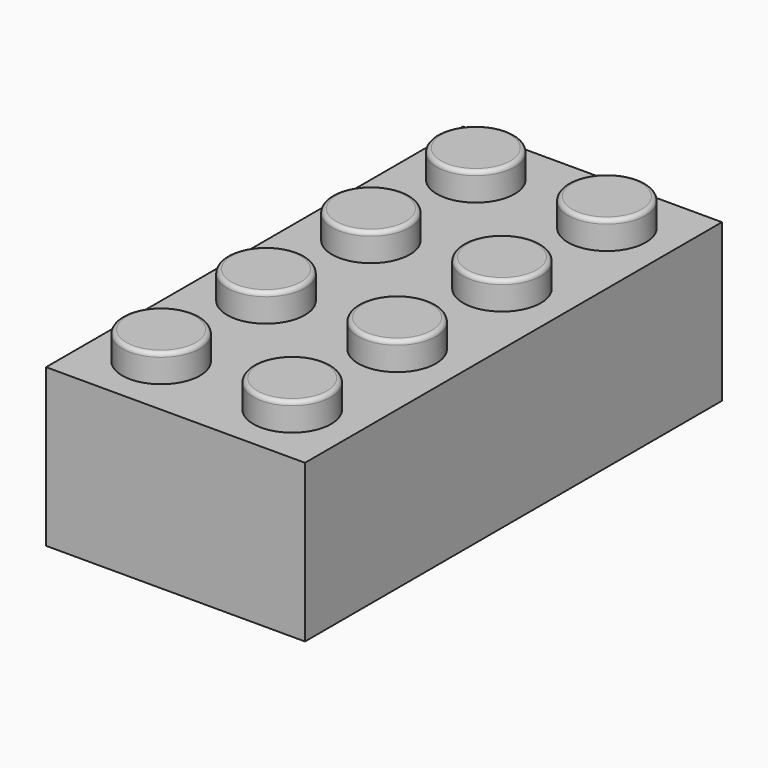
from build123d import *

# Parameters (mm, degrees)
F0_W      = 15.8
F0_H      = 31.8
F1_DEPTH  = 9.6
F2_R      = 2.3749
F3_DEPTH  = 1.7
F4_W      = 13.1584
F4_H      = 29.1584
F4_R      = 3.175
F5_DEPTH  = 8.763
F4_R_2    = 2.4892
F6_DEPTH  = 8.763
F8_DEPTH  = 6.477
F9_R      = 1.3
F10_DEPTH = 1.397
F11_R     = 0.254


# Not quite as in the source:
# - a feature names something its author has since deleted; it is built from what else it names


with BuildPart() as f1:
    # F0 (on Top) → F1 (new body)
    with BuildSketch(Plane.XY):
        with Locations((-7.9, -15.9)):
            Rectangle(F0_W, F0_H)
    extrude(amount=F1_DEPTH)

    # F2 (on face) → F3 (join)
    with BuildSketch(Plane.XY.offset(9.6)):
        with Locations((-3.9, -3.9)):
            Circle(F2_R)
        with Locations((-3.9, -11.9)):
            Circle(F2_R)
        with Locations((-3.9, -19.9)):
            Circle(F2_R)
        with Locations((-3.9, -27.9)):
            Circle(F2_R)
        with Locations((-11.9, -3.9)):
            Circle(F2_R)
        with Locations((-11.9, -11.9)):
            Circle(F2_R)
        with Locations((-11.9, -19.9)):
            Circle(F2_R)
        with Locations((-11.9, -27.9)):
            Circle(F2_R)
    extrude(amount=F3_DEPTH)

    # F4 (on face) → F5 (cut)
    with BuildSketch(Plane(origin=(0, 0, 0), x_dir=(1, 0, 0), z_dir=(0, 0, -1))):
        with Locations((-7.9, 15.9)):
            Rectangle(F4_W, F4_H)
        with Locations((-7.9, 7.9)):
            Circle(F4_R, mode=Mode.SUBTRACT)
        with Locations((-7.9, 15.9)):
            Circle(F4_R, mode=Mode.SUBTRACT)
        with Locations((-7.9, 23.9)):
            Circle(F4_R, mode=Mode.SUBTRACT)
    extrude(amount=-F5_DEPTH, mode=Mode.SUBTRACT)

    # F4 (on face) → F6 (cut)
    with BuildSketch(Plane(origin=(0, 0, 0), x_dir=(1, 0, 0), z_dir=(0, 0, -1))):
        with Locations((-7.9, 23.9)):
            Circle(F4_R_2)
        with Locations((-7.9, 15.9)):
            Circle(F4_R_2)
        with Locations((-7.9, 7.9)):
            Circle(F4_R_2)
    extrude(amount=-F6_DEPTH, mode=Mode.SUBTRACT)

    # F7 (on face) → F8 (join)
    with BuildSketch(Plane(origin=(0, 0, 8.763), x_dir=(1, 0, 0), z_dir=(0, 0, -1))):
        with BuildLine():
            Line((-1.3208, 16.3), (-4.7502976331, 16.3))
            ThreePointArc((-4.7502976331, 16.3), (-4.7313307198, 16.1003995822), (-4.725, 15.9))
            ThreePointArc((-4.725, 15.9), (-4.7313307198, 15.6996004178), (-4.7502976331, 15.5))
            Line((-4.7502976331, 15.5), (-1.3208, 15.5))
            Line((-1.3208, 15.5), (-1.3208, 16.3))
        make_face()
        with BuildLine():
            Line((-11.0497023669, 16.3), (-14.4792, 16.3))
            Line((-14.4792, 16.3), (-14.4792, 15.5))
            Line((-14.4792, 15.5), (-11.0497023669, 15.5))
            ThreePointArc((-11.0497023669, 15.5), (-11.075, 15.9), (-11.0497023669, 16.3))
        make_face()
    extrude(amount=F8_DEPTH)

    # F9 (on face) → F10 (cut)
    with BuildSketch(Plane(origin=(0, 0, 8.763), x_dir=(1, 0, 0), z_dir=(0, 0, -1))):
        with Locations((-11.9, 3.9)):
            Circle(F9_R)
        with Locations((-11.9, 11.9)):
            Circle(F9_R)
        with Locations((-11.9, 19.9)):
            Circle(F9_R)
        with Locations((-11.9, 27.9)):
            Circle(F9_R)
        with Locations((-3.9, 3.9)):
            Circle(F9_R)
        with Locations((-3.9, 11.9)):
            Circle(F9_R)
        with Locations((-3.9, 19.9)):
            Circle(F9_R)
        with Locations((-3.9, 27.9)):
            Circle(F9_R)
    extrude(amount=-F10_DEPTH, mode=Mode.SUBTRACT)

    # F11
    f11_edges = [f1.edges().sort_by_distance(p)[0] for p in [
        (-14.2749, -3.9, 11.3),
        (-6.2749, -3.9, 11.3),
        (-14.2749, -11.9, 11.3),
        (-14.2749, -19.9, 11.3),
        (-6.2749, -11.9, 11.3),
        (-6.2749, -19.9, 11.3),
        (-14.2749, -27.9, 11.3),
        (-6.2749, -27.9, 11.3),
    ]]
    fillet(f11_edges, radius=F11_R)


solid = f1.part
